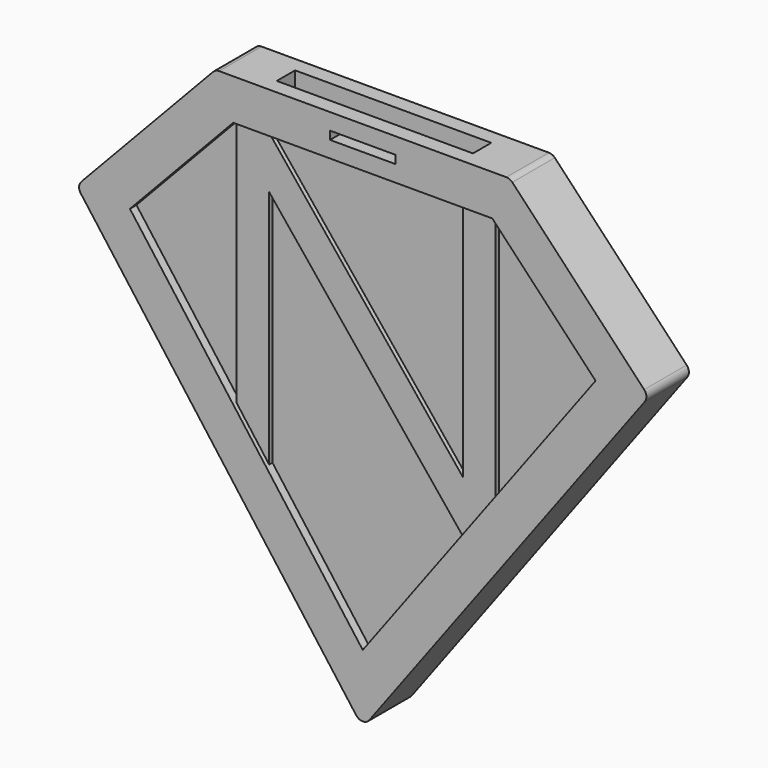
from build123d import *

# Parameters (mm, degrees)
F1_DEPTH  = 3.25
F3_DEPTH  = 0.5
F5_DEPTH  = 0.5
F7_DEPTH  = 0.5
F9_DEPTH  = 0.5
F10_W     = 24
F10_H     = 2.8
F11_DEPTH = 20
F13_DEPTH = 1.4
F14_W     = 8
F14_H     = 1
F15_DEPTH = 25
F16_R     = 1


# Not quite as in the source:
# - ends of sketch curves that miss each other by under 0.0002 mm in the source are joined


with BuildPart() as f1:
    # F0 (on Front) → F1 (new body, symmetric)
    with BuildSketch(Plane.XZ):
        Polygon((18, 18), (0, 18), (-18, 18), (-35, 0), (0, -47), (35, 0), align=None)
    extrude(amount=F1_DEPTH, both=True)

    # F2 (on face) → F3 (cut)
    with BuildSketch(Plane.XZ.offset(3.25)):
        Polygon((15.8447675538, 13), (-15.8447675538, 13), (-28.4822773709, -0.3808927475), (1.162e-07, -38.628522516), (28.4822775009, -0.3808928851), align=None)
    extrude(amount=-F3_DEPTH, mode=Mode.SUBTRACT)

    # F4 (on face) → F5 (cut)
    with BuildSketch(Plane(origin=(0, 3.25, 0), x_dir=(-1, 0, 0), z_dir=(0, 1, 0))):
        Polygon((28.482277527, -0.3808925379), (15.8447676545, 13.0000002682), (-15.8447670441, 13.0000002682), (-28.4822772579, -0.3808928993), (0, -38.6285223599), align=None)
    extrude(amount=-F5_DEPTH, mode=Mode.SUBTRACT)

    # F6 (on face) → F7 (cut)
    with BuildSketch(Plane.XZ.offset(2.75)):
        Polygon((-15.8447675538, -17.3512630734), (-15.8447675538, 13), (-28.4822773709, -0.3808927475), align=None)
        Polygon((28.4822775009, -0.3808928851), (15.8447675538, 13), (15.8447675538, -17.3512633855), align=None)
        Polygon((11.8447675538, -22.7226919569), (-11.8447675538, 6.6308805462), (-11.8447675538, -22.7226916448), (1.162e-07, -38.628522516), align=None)
        Polygon((11.8447675538, -16.3535725031), (11.8447675538, 13), (-11.8447675538, 13), align=None)
    extrude(amount=-F7_DEPTH, mode=Mode.SUBTRACT)

    # F8 (on face) → F9 (cut)
    with BuildSketch(Plane(origin=(0, 2.75, 0), x_dir=(-1, 0, 0), z_dir=(0, 1, 0))):
        Polygon((-15.8447675538, -17.3512633855), (-15.8447675538, 13), (-28.4822772579, -0.3808928993), align=None)
        Polygon((28.482277527, -0.3808925379), (15.8447676545, 13.0000002682), (15.8447675538, -17.3512630734), align=None)
        Polygon((11.8447675538, -16.353572196), (11.8447675538, 13.0000002682), (-11.8447675538, 13.0000002682), align=None)
        Polygon((0, -38.6285223599), (11.8447675538, -22.7226916448), (-11.8447675538, 6.6308808195), (-11.8447675538, -22.7226916448), align=None)
    extrude(amount=-F9_DEPTH, mode=Mode.SUBTRACT)

    # F10 (on face) → F11 (cut)
    with BuildSketch(Plane.XY.offset(18)):
        Rectangle(F10_W, F10_H)
    extrude(amount=-F11_DEPTH, mode=Mode.SUBTRACT)

    # F12 (on Front) → F13 (cut, symmetric)
    with BuildSketch(Plane.XZ):
        with BuildLine():
            Line((12, -2), (-12, -2))
            ThreePointArc((-12, -2), (0, -14), (12, -2))
        make_face()
    extrude(amount=F13_DEPTH, both=True, mode=Mode.SUBTRACT)

    # F14 (on face) → F15 (cut)
    with BuildSketch(Plane.XZ.offset(3.25)):
        with Locations((0, 15.5)):
            Rectangle(F14_W, F14_H)
    extrude(amount=-F15_DEPTH, mode=Mode.SUBTRACT)

    # F16
    f16_edges = [f1.edges().sort_by_distance(p)[0] for p in [
        (0, 0, -47),
        (35, 0, 0),
        (-35, 0, 0),
        (-18, 0, 18),
        (18, 0, 18),
    ]]
    fillet(f16_edges, radius=F16_R)


solid = f1.part
